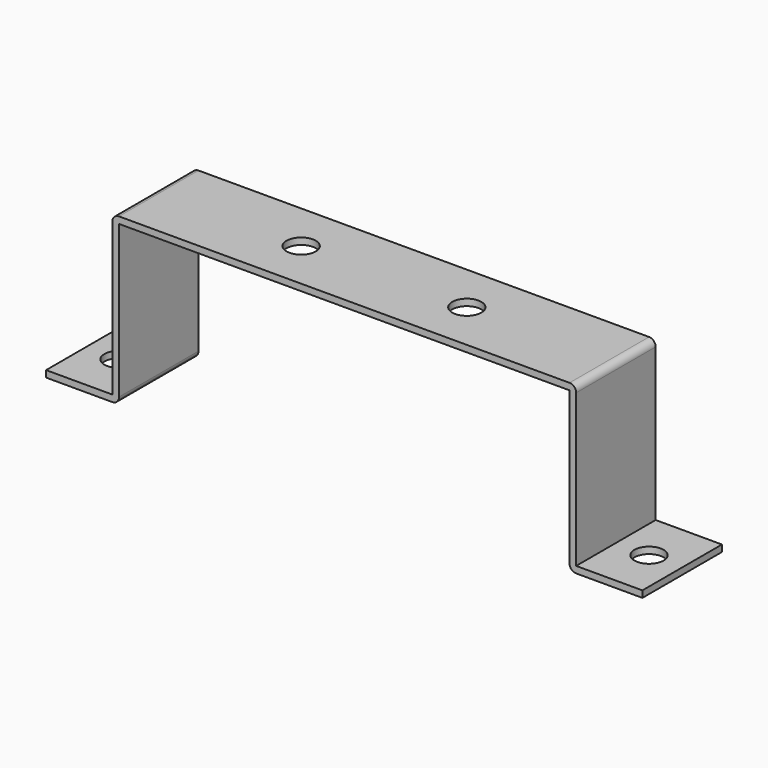
from build123d import *

# Parameters (mm, degrees)
F1_DEPTH = 30
F2_R     = 4.4
F3_R     = 4.4
F4_DEPTH = 25
F5_R     = 2
F6_R     = 2


# Not quite as in the source:
# - a feature names something its author has since deleted; it is built from what else it names


with BuildPart() as f1:
    # F0 (on Front) → F1 (new body)
    with BuildSketch(Plane.XZ):
        Polygon((90, -1), (90, 1), (70, 1), (70, 49), (-70, 49), (-70, 1), (-90, 1), (-90, -1), (-68, -1), (-68, 47), (68, 47), (68, -1), align=None)
    extrude(amount=F1_DEPTH)

    # F2 (on face) + F3 (on face) → F4 (cut)
    with BuildSketch(Plane.XY.offset(1)):
        with Locations((-80, -15)):
            Circle(F2_R)
        with Locations((80, -15)):
            Circle(F2_R)
    with BuildSketch(Plane.XY.offset(49)):
        with Locations((-25, -15)):
            Circle(F3_R)
        with Locations((25, -15)):
            Circle(F3_R)
    extrude(amount=-F4_DEPTH, mode=Mode.SUBTRACT)

    # F5
    f5_edges = [f1.edges().sort_by_distance(p)[0] for p in [
        (-70, -15, 49),
        (70, -15, 49),
    ]]
    fillet(f5_edges, radius=F5_R)

    # F6
    f6_edges = [f1.edges().sort_by_distance(p)[0] for p in [
        (68, -15, -1),
        (-68, -15, -1),
    ]]
    fillet(f6_edges, radius=F6_R)


solid = f1.part
